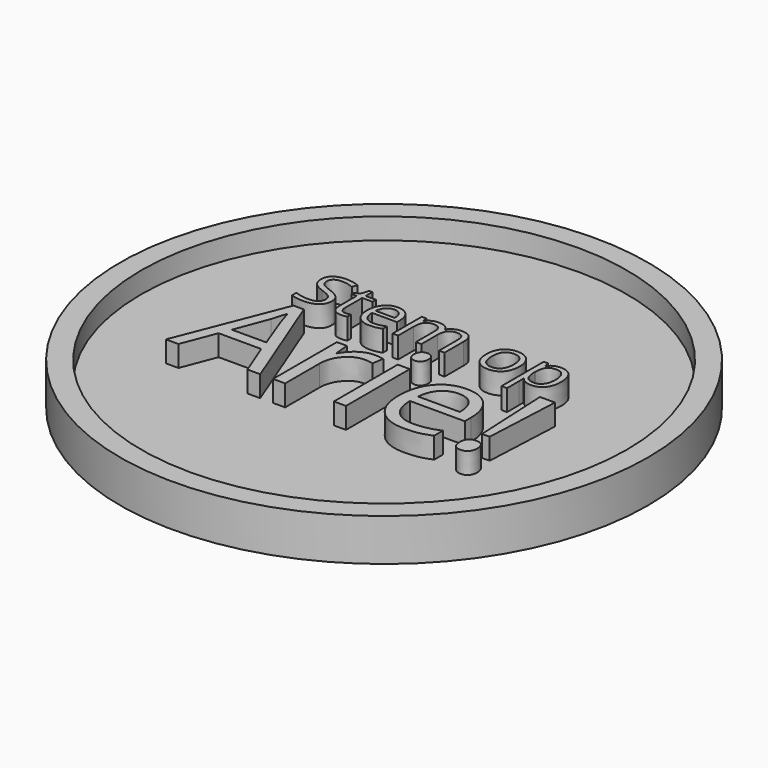
from build123d import *

# Parameters (mm, degrees)
F0_R           = 25
F0_R_2         = 23
F0_TEXT_SIZE   = 6.4365281206
F0_TEXT_SIZE_2 = 14.1188372961
F1_DEPTH       = 4
F0_W           = 1.144949462
F0_H           = 7.5557840218
F2_DEPTH       = 2


# Not quite as in the source:
# - Text() gives the source's letters only with a copy of the font that has no kerning and outlines rounded to 1/6400 em; it was checked with that copy


with BuildPart() as f1:
    # F0 (on Top) → F1 (new body)
    with BuildSketch(Plane.XY):
        with Locations((-25.1149237156, 15.8463213593)):
            Circle(F0_R)
        with Locations((-25.1149237156, 15.8463213593)):
            Circle(F0_R_2, mode=Mode.SUBTRACT)
        with Locations((-37.2358597815, 19.5541195571)):
            Text('Stem op', F0_TEXT_SIZE, font='Open Sans', text_align=(TextAlign.LEFT, TextAlign.BOTTOM))
        with Locations((-39.7772528231, 8.3421012387)):
            Text('Arie!', F0_TEXT_SIZE_2, font='Open Sans', text_align=(TextAlign.LEFT, TextAlign.BOTTOM))
    extrude(amount=F1_DEPTH)

    # F0 (on Top) → F2 (join)
    with BuildSketch(Plane.XY):
        with Locations((-25.1149237156, 15.8463213593)):
            Circle(F0_R_2)
        Polygon((-30.8426760967, 8.3421012387), (-32.0560136768, 8.3421012387), (-33.3112665552, 11.5475185186), (-37.3505776628, 11.5475185186), (-38.5903880629, 8.3421012387), (-39.7772528231, 8.3421012387), (-35.7930934236, 18.4635427253), (-34.8069808812, 18.4635427253), align=None, mode=Mode.SUBTRACT)
        with BuildLine():
            add(Edge.make_bspline(
                [(-27.4850401022, 15.6364661636), (-26.8916077221, 16.0368675651), (-26.1812537206, 16.0368675651)],
                knots=[0, 0, 0, 1, 1, 1], degree=2))
            add(Edge.make_bspline(
                [(-26.1812537206, 16.0368675651), (-25.6782701419, 16.0368675651), (-25.2789717746, 15.9530369686)],
                knots=[0, 0, 0, 1, 1, 1], degree=2))
            Line((-25.2789717746, 15.9530369686), (-25.4378086942, 14.8919181031))
            add(Edge.make_bspline(
                [(-25.4378086942, 14.8919181031), (-25.9054951797, 14.9956033145), (-26.265084317, 14.9956033145)],
                knots=[0, 0, 0, 1, 1, 1], degree=2))
            add(Edge.make_bspline(
                [(-26.265084317, 14.9956033145), (-27.1828087413, 14.9956033145), (-27.8335988979, 14.2510552539)],
                knots=[0, 0, 0, 1, 1, 1], degree=2))
            add(Edge.make_bspline(
                [(-27.8335988979, 14.2510552539), (-28.4843890545, 13.5065071934), (-28.4843890545, 12.3968548247)],
                knots=[0, 0, 0, 1, 1, 1], degree=2))
            Line((-28.4843890545, 12.3968548247), (-28.4843890545, 8.3421012387))
            Line((-28.4843890545, 8.3421012387), (-29.6293385165, 8.3421012387))
            Line((-29.6293385165, 8.3421012387), (-29.6293385165, 15.8978852604))
            Line((-29.6293385165, 15.8978852604), (-28.6851412723, 15.8978852604))
            Line((-28.6851412723, 15.8978852604), (-28.5527771727, 14.4992379408))
            Line((-28.5527771727, 14.4992379408), (-28.4976254645, 14.4992379408))
            add(Edge.make_bspline(
                [(-28.4976254645, 14.4992379408), (-28.0784724823, 15.2360647622), (-27.4850401022, 15.6364661636)],
                knots=[0, 0, 0, 1, 1, 1], degree=2))
        make_face(mode=Mode.SUBTRACT)
        with Locations((-23.2924072457, 12.1199932495)):
            Rectangle(F0_W, F0_H, mode=Mode.SUBTRACT)
        with BuildLine():
            add(Edge.make_bspline(
                [(-15.7950840346, 8.3178344871), (-16.3355707749, 8.203118934), (-17.1010764845, 8.203118934)],
                knots=[0, 0, 0, 1, 1, 1], degree=2))
            add(Edge.make_bspline(
                [(-17.1010764845, 8.203118934), (-18.7754823451, 8.203118934), (-19.7450493751, 9.2245285697)],
                knots=[0, 0, 0, 1, 1, 1], degree=2))
            add(Edge.make_bspline(
                [(-19.7450493751, 9.2245285697), (-20.714616405, 10.2459382053), (-20.714616405, 12.0571203022)],
                knots=[0, 0, 0, 1, 1, 1], degree=2))
            add(Edge.make_bspline(
                [(-20.714616405, 12.0571203022), (-20.714616405, 13.8859509457), (-19.8145405274, 14.9614092554)],
                knots=[0, 0, 0, 1, 1, 1], degree=2))
            add(Edge.make_bspline(
                [(-19.8145405274, 14.9614092554), (-18.9144646497, 16.0368675651), (-17.3966896404, 16.0368675651)],
                knots=[0, 0, 0, 1, 1, 1], degree=2))
            add(Edge.make_bspline(
                [(-17.3966896404, 16.0368675651), (-15.9781877058, 16.0368675651), (-15.150912083, 15.1025976284)],
                knots=[0, 0, 0, 1, 1, 1], degree=2))
            add(Edge.make_bspline(
                [(-15.150912083, 15.1025976284), (-14.3236364602, 14.1683276917), (-14.3236364602, 12.6373162724)],
                knots=[0, 0, 0, 1, 1, 1], degree=2))
            Line((-14.3236364602, 12.6373162724), (-14.3236364602, 11.9137258609))
            Line((-14.3236364602, 11.9137258609), (-19.5277516448, 11.9137258609))
            add(Edge.make_bspline(
                [(-19.5277516448, 11.9137258609), (-19.4924545516, 10.5834666594), (-18.8549008049, 9.8940703071)],
                knots=[0, 0, 0, 1, 1, 1], degree=2))
            add(Edge.make_bspline(
                [(-18.8549008049, 9.8940703071), (-18.2173470583, 9.2046739547), (-17.0591611863, 9.2046739547)],
                knots=[0, 0, 0, 1, 1, 1], degree=2))
            add(Edge.make_bspline(
                [(-17.0591611863, 9.2046739547), (-15.8392054012, 9.2046739547), (-14.6479285043, 9.7142757384)],
                knots=[0, 0, 0, 1, 1, 1], degree=2))
            Line((-14.6479285043, 9.7142757384), (-14.6479285043, 8.6928661027))
            add(Edge.make_bspline(
                [(-14.6479285043, 8.6928661027), (-15.2545972944, 8.4325500401), (-15.7950840346, 8.3178344871)],
                knots=[0, 0, 0, 1, 1, 1], degree=2))
        make_face(mode=Mode.SUBTRACT)
        with BuildLine():
            add(Edge.make_bspline(
                [(-12.301774838, 8.3586467511), (-12.5367211149, 8.5759444814), (-12.5367211149, 9.0723098551)],
                knots=[0, 0, 0, 1, 1, 1], degree=2))
            add(Edge.make_bspline(
                [(-12.5367211149, 9.0723098551), (-12.5367211149, 10.0098888943), (-11.7094454921, 10.0098888943)],
                knots=[0, 0, 0, 1, 1, 1], degree=2))
            add(Edge.make_bspline(
                [(-11.7094454921, 10.0098888943), (-11.3101471248, 10.0098888943), (-11.0928493945, 9.7694274466)],
                knots=[0, 0, 0, 1, 1, 1], degree=2))
            add(Edge.make_bspline(
                [(-11.0928493945, 9.7694274466), (-10.8755516643, 9.5289659989), (-10.8755516643, 9.0723098551)],
                knots=[0, 0, 0, 1, 1, 1], degree=2))
            add(Edge.make_bspline(
                [(-10.8755516643, 9.0723098551), (-10.8755516643, 8.6310961896), (-11.096158497, 8.3862226052)],
                knots=[0, 0, 0, 1, 1, 1], degree=2))
            add(Edge.make_bspline(
                [(-11.096158497, 8.3862226052), (-11.3167653298, 8.1413490209), (-11.7094454921, 8.1413490209)],
                knots=[0, 0, 0, 1, 1, 1], degree=2))
            add(Edge.make_bspline(
                [(-11.7094454921, 8.1413490209), (-12.0668285611, 8.1413490209), (-12.301774838, 8.3586467511)],
                knots=[0, 0, 0, 1, 1, 1], degree=2))
        make_face(mode=Mode.SUBTRACT)
        Polygon((-10.9858550806, 18.4216274271), (-11.3366199447, 11.119541263), (-12.0602103561, 11.119541263), (-12.4131812885, 18.4216274271), align=None, mode=Mode.SUBTRACT)
        with BuildLine():
            add(Edge.make_bspline(
                [(-34.2831025062, 21.5434090294), (-34.0115614761, 21.2477310189), (-34.0115614761, 20.7770599001)],
                knots=[0, 0, 0, 1, 1, 1], degree=2))
            add(Edge.make_bspline(
                [(-34.0115614761, 20.7770599001), (-34.0115614761, 20.1706182662), (-34.4515585156, 19.8306891248)],
                knots=[0, 0, 0, 1, 1, 1], degree=2))
            add(Edge.make_bspline(
                [(-34.4515585156, 19.8306891248), (-34.8915555551, 19.4907599835), (-35.6458361942, 19.4907599835)],
                knots=[0, 0, 0, 1, 1, 1], degree=2))
            add(Edge.make_bspline(
                [(-35.6458361942, 19.4907599835), (-36.4624706995, 19.4907599835), (-36.9029705928, 19.7019585624)],
                knots=[0, 0, 0, 1, 1, 1], degree=2))
            Line((-36.9029705928, 19.7019585624), (-36.9029705928, 20.2168808121))
            add(Edge.make_bspline(
                [(-36.9029705928, 20.2168808121), (-36.6193610725, 20.0982073248), (-36.2864718837, 20.028813506)],
                knots=[0, 0, 0, 1, 1, 1], degree=2))
            add(Edge.make_bspline(
                [(-36.2864718837, 20.028813506), (-35.953582695, 19.9594196872), (-35.6267277514, 19.9594196872)],
                knots=[0, 0, 0, 1, 1, 1], degree=2))
            add(Edge.make_bspline(
                [(-35.6267277514, 19.9594196872), (-35.0926970588, 19.9594196872), (-34.8221617363, 20.1620697523)],
                knots=[0, 0, 0, 1, 1, 1], degree=2))
            add(Edge.make_bspline(
                [(-34.8221617363, 20.1620697523), (-34.5516264137, 20.3647198173), (-34.5516264137, 20.7267745241)],
                knots=[0, 0, 0, 1, 1, 1], degree=2))
            add(Edge.make_bspline(
                [(-34.5516264137, 20.7267745241), (-34.5516264137, 20.9651272061), (-34.6476714818, 21.1174918952)],
                knots=[0, 0, 0, 1, 1, 1], degree=2))
            add(Edge.make_bspline(
                [(-34.6476714818, 21.1174918952), (-34.7437165498, 21.2698565843), (-34.9684921803, 21.3990900005)],
                knots=[0, 0, 0, 1, 1, 1], degree=2))
            add(Edge.make_bspline(
                [(-34.9684921803, 21.3990900005), (-35.1932678107, 21.5283234166), (-35.6518704393, 21.6912480347)],
                knots=[0, 0, 0, 1, 1, 1], degree=2))
            add(Edge.make_bspline(
                [(-35.6518704393, 21.6912480347), (-36.2925061288, 21.920549349), (-36.5675671352, 22.2348329486)],
                knots=[0, 0, 0, 1, 1, 1], degree=2))
            add(Edge.make_bspline(
                [(-36.5675671352, 22.2348329486), (-36.8426281416, 22.5491165483), (-36.8426281416, 23.0549874302)],
                knots=[0, 0, 0, 1, 1, 1], degree=2))
            add(Edge.make_bspline(
                [(-36.8426281416, 23.0549874302), (-36.8426281416, 23.5860010002), (-36.4438651104, 23.9002845998)],
                knots=[0, 0, 0, 1, 1, 1], degree=2))
            add(Edge.make_bspline(
                [(-36.4438651104, 23.9002845998), (-36.0451020792, 24.2145681995), (-35.3873693619, 24.2145681995)],
                knots=[0, 0, 0, 1, 1, 1], degree=2))
            add(Edge.make_bspline(
                [(-35.3873693619, 24.2145681995), (-34.7024825415, 24.2145681995), (-34.1272178408, 23.9631413198)],
                knots=[0, 0, 0, 1, 1, 1], degree=2))
            Line((-34.1272178408, 23.9631413198), (-34.2941652889, 23.498504446))
            add(Edge.make_bspline(
                [(-34.2941652889, 23.498504446), (-34.8633957445, 23.736857128), (-35.4004435596, 23.736857128)],
                knots=[0, 0, 0, 1, 1, 1], degree=2))
            add(Edge.make_bspline(
                [(-35.4004435596, 23.736857128), (-35.8248521326, 23.736857128), (-36.0637076683, 23.5548240671)],
                knots=[0, 0, 0, 1, 1, 1], degree=2))
            add(Edge.make_bspline(
                [(-36.0637076683, 23.5548240671), (-36.302563204, 23.3727910062), (-36.302563204, 23.0489531851)],
                knots=[0, 0, 0, 1, 1, 1], degree=2))
            add(Edge.make_bspline(
                [(-36.302563204, 23.0489531851), (-36.302563204, 22.8106005032), (-36.2145637961, 22.6577329603)],
                knots=[0, 0, 0, 1, 1, 1], degree=2))
            add(Edge.make_bspline(
                [(-36.2145637961, 22.6577329603), (-36.1265643882, 22.5048654174), (-35.9173772243, 22.3776434163)],
                knots=[0, 0, 0, 1, 1, 1], degree=2))
            add(Edge.make_bspline(
                [(-35.9173772243, 22.3776434163), (-35.7081900604, 22.2504214152), (-35.2777472423, 22.0965481648)],
                knots=[0, 0, 0, 1, 1, 1], degree=2))
            add(Edge.make_bspline(
                [(-35.2777472423, 22.0965481648), (-34.5546435363, 21.83908704), (-34.2831025062, 21.5434090294)],
                knots=[0, 0, 0, 1, 1, 1], degree=2))
        make_face(mode=Mode.SUBTRACT)
        with BuildLine():
            add(Edge.make_bspline(
                [(-32.4426577467, 20.0886531034), (-32.2948187414, 19.922208509), (-32.0373576166, 19.922208509)],
                knots=[0, 0, 0, 1, 1, 1], degree=2))
            add(Edge.make_bspline(
                [(-32.0373576166, 19.922208509), (-31.898569979, 19.922208509), (-31.7698394166, 19.9423226594)],
                knots=[0, 0, 0, 1, 1, 1], degree=2))
            add(Edge.make_bspline(
                [(-31.7698394166, 19.9423226594), (-31.6411088542, 19.9624368098), (-31.5656807903, 19.9845623752)],
                knots=[0, 0, 0, 1, 1, 1], degree=2))
            Line((-31.5656807903, 19.9845623752), (-31.5656807903, 19.5852964902))
            add(Edge.make_bspline(
                [(-31.5656807903, 19.5852964902), (-31.6501602218, 19.5450681895), (-31.8150962549, 19.5179140865)],
                knots=[0, 0, 0, 1, 1, 1], degree=2))
            add(Edge.make_bspline(
                [(-31.8150962549, 19.5179140865), (-31.980032288, 19.4907599835), (-32.1127856805, 19.4907599835)],
                knots=[0, 0, 0, 1, 1, 1], degree=2))
            add(Edge.make_bspline(
                [(-32.1127856805, 19.4907599835), (-33.1114532467, 19.4907599835), (-33.1114532467, 20.5437357557)],
                knots=[0, 0, 0, 1, 1, 1], degree=2))
            Line((-33.1114532467, 20.5437357557), (-33.1114532467, 22.5933676791))
            Line((-33.1114532467, 22.5933676791), (-33.6052556385, 22.5933676791))
            Line((-33.6052556385, 22.5933676791), (-33.6052556385, 22.8447945588))
            Line((-33.6052556385, 22.8447945588), (-33.1114532467, 23.0620273829))
            Line((-33.1114532467, 23.0620273829), (-32.8922090076, 23.7971995791))
            Line((-32.8922090076, 23.7971995791), (-32.590496752, 23.7971995791))
            Line((-32.590496752, 23.7971995791), (-32.590496752, 22.9986678092))
            Line((-32.590496752, 22.9986678092), (-31.5908234782, 22.9986678092))
            Line((-31.5908234782, 22.9986678092), (-31.5908234782, 22.5933676791))
            Line((-31.5908234782, 22.5933676791), (-32.590496752, 22.5933676791))
            Line((-32.590496752, 22.5933676791), (-32.590496752, 20.5658613211))
            add(Edge.make_bspline(
                [(-32.590496752, 20.5658613211), (-32.590496752, 20.2550976978), (-32.4426577467, 20.0886531034)],
                knots=[0, 0, 0, 1, 1, 1], degree=2))
        make_face(mode=Mode.SUBTRACT)
        with BuildLine():
            add(Edge.make_bspline(
                [(-28.8271392164, 19.5430567744), (-29.0735375586, 19.4907599835), (-29.4225180676, 19.4907599835)],
                knots=[0, 0, 0, 1, 1, 1], degree=2))
            add(Edge.make_bspline(
                [(-29.4225180676, 19.4907599835), (-30.1858500744, 19.4907599835), (-30.6278585289, 19.9564025647)],
                knots=[0, 0, 0, 1, 1, 1], degree=2))
            add(Edge.make_bspline(
                [(-30.6278585289, 19.9564025647), (-31.0698669835, 20.4220451459), (-31.0698669835, 21.2477310189)],
                knots=[0, 0, 0, 1, 1, 1], degree=2))
            add(Edge.make_bspline(
                [(-31.0698669835, 21.2477310189), (-31.0698669835, 22.081462552), (-30.6595383158, 22.5717449674)],
                knots=[0, 0, 0, 1, 1, 1], degree=2))
            add(Edge.make_bspline(
                [(-30.6595383158, 22.5717449674), (-30.2492096481, 23.0620273829), (-29.5572828751, 23.0620273829)],
                knots=[0, 0, 0, 1, 1, 1], degree=2))
            add(Edge.make_bspline(
                [(-29.5572828751, 23.0620273829), (-28.9106129405, 23.0620273829), (-28.5334726209, 22.6361102486)],
                knots=[0, 0, 0, 1, 1, 1], degree=2))
            add(Edge.make_bspline(
                [(-28.5334726209, 22.6361102486), (-28.1563323014, 22.2101931144), (-28.1563323014, 21.5122320963)],
                knots=[0, 0, 0, 1, 1, 1], degree=2))
            Line((-28.1563323014, 21.5122320963), (-28.1563323014, 21.1823600302))
            Line((-28.1563323014, 21.1823600302), (-30.5287963383, 21.1823600302))
            add(Edge.make_bspline(
                [(-30.5287963383, 21.1823600302), (-30.512705018, 20.5759183963), (-30.2220555451, 20.2616347966)],
                knots=[0, 0, 0, 1, 1, 1], degree=2))
            add(Edge.make_bspline(
                [(-30.2220555451, 20.2616347966), (-29.9314060721, 19.947351197), (-29.4034096247, 19.947351197)],
                knots=[0, 0, 0, 1, 1, 1], degree=2))
            add(Edge.make_bspline(
                [(-29.4034096247, 19.947351197), (-28.8472533668, 19.947351197), (-28.3041713066, 20.1796696339)],
                knots=[0, 0, 0, 1, 1, 1], degree=2))
            Line((-28.3041713066, 20.1796696339), (-28.3041713066, 19.7140270526))
            add(Edge.make_bspline(
                [(-28.3041713066, 19.7140270526), (-28.5807408743, 19.5953535654), (-28.8271392164, 19.5430567744)],
                knots=[0, 0, 0, 1, 1, 1], degree=2))
        make_face(mode=Mode.SUBTRACT)
        with BuildLine():
            add(Edge.make_bspline(
                [(-23.7689180045, 17.3693328349), (-23.9619489831, 17.5590547111), (-23.9619489831, 17.9451166684)],
                knots=[0, 0, 0, 1, 1, 1], degree=2))
            add(Edge.make_bspline(
                [(-23.9619489831, 17.9451166684), (-23.9619489831, 18.3377968307), (-23.7689180045, 18.5209005019)],
                knots=[0, 0, 0, 1, 1, 1], degree=2))
            add(Edge.make_bspline(
                [(-23.7689180045, 18.5209005019), (-23.5758870258, 18.704004173), (-23.2846860066, 18.704004173)],
                knots=[0, 0, 0, 1, 1, 1], degree=2))
            add(Edge.make_bspline(
                [(-23.2846860066, 18.704004173), (-23.0089274656, 18.704004173), (-22.809278282, 18.5175913994)],
                knots=[0, 0, 0, 1, 1, 1], degree=2))
            add(Edge.make_bspline(
                [(-22.809278282, 18.5175913994), (-22.6096290983, 18.3311786257), (-22.6096290983, 17.9451166684)],
                knots=[0, 0, 0, 1, 1, 1], degree=2))
            add(Edge.make_bspline(
                [(-22.6096290983, 17.9451166684), (-22.6096290983, 17.5590547111), (-22.809278282, 17.3693328349)],
                knots=[0, 0, 0, 1, 1, 1], degree=2))
            add(Edge.make_bspline(
                [(-22.809278282, 17.3693328349), (-23.0089274656, 17.1796109587), (-23.2846860066, 17.1796109587)],
                knots=[0, 0, 0, 1, 1, 1], degree=2))
            add(Edge.make_bspline(
                [(-23.2846860066, 17.1796109587), (-23.5758870258, 17.1796109587), (-23.7689180045, 17.3693328349)],
                knots=[0, 0, 0, 1, 1, 1], degree=2))
        make_face(mode=Mode.SUBTRACT)
        with BuildLine():
            Line((-22.3544056252, 19.5541195571), (-22.8753621199, 19.5541195571))
            Line((-22.8753621199, 19.5541195571), (-22.8753621199, 21.7948359091))
            add(Edge.make_bspline(
                [(-22.8753621199, 21.7948359091), (-22.8753621199, 22.2071759919), (-23.0513609357, 22.4128431795)],
                knots=[0, 0, 0, 1, 1, 1], degree=2))
            add(Edge.make_bspline(
                [(-23.0513609357, 22.4128431795), (-23.2273597515, 22.6185103671), (-23.598465826, 22.6185103671)],
                knots=[0, 0, 0, 1, 1, 1], degree=2))
            add(Edge.make_bspline(
                [(-23.598465826, 22.6185103671), (-24.0852282651, 22.6185103671), (-24.3180495557, 22.3389236768)],
                knots=[0, 0, 0, 1, 1, 1], degree=2))
            add(Edge.make_bspline(
                [(-24.3180495557, 22.3389236768), (-24.5508708463, 22.0593369866), (-24.5508708463, 21.4780380407)],
                knots=[0, 0, 0, 1, 1, 1], degree=2))
            Line((-24.5508708463, 21.4780380407), (-24.5508708463, 19.5541195571))
            Line((-24.5508708463, 19.5541195571), (-25.0728330486, 19.5541195571))
            Line((-25.0728330486, 19.5541195571), (-25.0728330486, 21.7948359091))
            add(Edge.make_bspline(
                [(-25.0728330486, 21.7948359091), (-25.0728330486, 22.2071759919), (-25.2488318644, 22.4128431795)],
                knots=[0, 0, 0, 1, 1, 1], degree=2))
            add(Edge.make_bspline(
                [(-25.2488318644, 22.4128431795), (-25.4248306802, 22.6185103671), (-25.7989538772, 22.6185103671)],
                knots=[0, 0, 0, 1, 1, 1], degree=2))
            add(Edge.make_bspline(
                [(-25.7989538772, 22.6185103671), (-26.2887334389, 22.6185103671), (-26.5165261919, 22.3248437716)],
                knots=[0, 0, 0, 1, 1, 1], degree=2))
            add(Edge.make_bspline(
                [(-26.5165261919, 22.3248437716), (-26.7443189449, 22.0311771761), (-26.7443189449, 21.3613759685)],
                knots=[0, 0, 0, 1, 1, 1], degree=2))
            Line((-26.7443189449, 21.3613759685), (-26.7443189449, 19.5541195571))
            Line((-26.7443189449, 19.5541195571), (-27.2662811472, 19.5541195571))
            Line((-27.2662811472, 19.5541195571), (-27.2662811472, 22.9986678092))
            Line((-27.2662811472, 22.9986678092), (-26.8418725742, 22.9986678092))
            Line((-26.8418725742, 22.9986678092), (-26.7573931427, 22.5269909828))
            Line((-26.7573931427, 22.5269909828), (-26.7322504547, 22.5269909828))
            add(Edge.make_bspline(
                [(-26.7322504547, 22.5269909828), (-26.5844114494, 22.7784178626), (-26.3153846881, 22.9202226227)],
                knots=[0, 0, 0, 1, 1, 1], degree=2))
            add(Edge.make_bspline(
                [(-26.3153846881, 22.9202226227), (-26.0463579268, 23.0620273829), (-25.7134687381, 23.0620273829)],
                knots=[0, 0, 0, 1, 1, 1], degree=2))
            add(Edge.make_bspline(
                [(-25.7134687381, 23.0620273829), (-24.9058856005, 23.0620273829), (-24.6574758433, 22.4767056069)],
                knots=[0, 0, 0, 1, 1, 1], degree=2))
            Line((-24.6574758433, 22.4767056069), (-24.6323331553, 22.4767056069))
            add(Edge.make_bspline(
                [(-24.6323331553, 22.4767056069), (-24.478459905, 22.7472409295), (-24.1863018707, 22.9046341562)],
                knots=[0, 0, 0, 1, 1, 1], degree=2))
            add(Edge.make_bspline(
                [(-24.1863018707, 22.9046341562), (-23.8941438365, 23.0620273829), (-23.5200206395, 23.0620273829)],
                knots=[0, 0, 0, 1, 1, 1], degree=2))
            add(Edge.make_bspline(
                [(-23.5200206395, 23.0620273829), (-22.9357045711, 23.0620273829), (-22.6450550981, 22.7618236885)],
                knots=[0, 0, 0, 1, 1, 1], degree=2))
            add(Edge.make_bspline(
                [(-22.6450550981, 22.7618236885), (-22.3544056252, 22.4616199941), (-22.3544056252, 21.8008701542)],
                knots=[0, 0, 0, 1, 1, 1], degree=2))
            Line((-22.3544056252, 21.8008701542), (-22.3544056252, 19.5541195571))
        make_face(mode=Mode.SUBTRACT)
        with BuildLine():
            add(Edge.make_bspline(
                [(-17.0598583922, 22.5807963351), (-16.633941258, 22.0995652873), (-16.633941258, 21.2799136595)],
                knots=[0, 0, 0, 1, 1, 1], degree=2))
            add(Edge.make_bspline(
                [(-16.633941258, 21.2799136595), (-16.633941258, 20.4371307587), (-17.0578469772, 19.9639453711)],
                knots=[0, 0, 0, 1, 1, 1], degree=2))
            add(Edge.make_bspline(
                [(-17.0578469772, 19.9639453711), (-17.4817526964, 19.4907599835), (-18.2299990904, 19.4907599835)],
                knots=[0, 0, 0, 1, 1, 1], degree=2))
            add(Edge.make_bspline(
                [(-18.2299990904, 19.4907599835), (-18.6926245491, 19.4907599835), (-19.0506564258, 19.7079928075)],
                knots=[0, 0, 0, 1, 1, 1], degree=2))
            add(Edge.make_bspline(
                [(-19.0506564258, 19.7079928075), (-19.4086883025, 19.9252256316), (-19.6037955611, 20.3305257617)],
                knots=[0, 0, 0, 1, 1, 1], degree=2))
            add(Edge.make_bspline(
                [(-19.6037955611, 20.3305257617), (-19.7989028198, 20.7358258918), (-19.7989028198, 21.2799136595)],
                knots=[0, 0, 0, 1, 1, 1], degree=2))
            add(Edge.make_bspline(
                [(-19.7989028198, 21.2799136595), (-19.7989028198, 22.1216908528), (-19.3775113694, 22.5918591178)],
                knots=[0, 0, 0, 1, 1, 1], degree=2))
            add(Edge.make_bspline(
                [(-19.3775113694, 22.5918591178), (-18.956119919, 23.0620273829), (-18.207873525, 23.0620273829)],
                knots=[0, 0, 0, 1, 1, 1], degree=2))
            add(Edge.make_bspline(
                [(-18.207873525, 23.0620273829), (-17.4857755264, 23.0620273829), (-17.0598583922, 22.5807963351)],
                knots=[0, 0, 0, 1, 1, 1], degree=2))
        make_face(mode=Mode.SUBTRACT)
        with BuildLine():
            add(Edge.make_bspline(
                [(-13.0641824198, 19.9609282485), (-13.4428313007, 19.4907599835), (-14.1156496308, 19.4907599835)],
                knots=[0, 0, 0, 1, 1, 1], degree=2))
            add(Edge.make_bspline(
                [(-14.1156496308, 19.4907599835), (-14.4525616496, 19.4907599835), (-14.7306397786, 19.614964862)],
                knots=[0, 0, 0, 1, 1, 1], degree=2))
            add(Edge.make_bspline(
                [(-14.7306397786, 19.614964862), (-15.0087179075, 19.7391697406), (-15.1967852135, 19.997636573)],
                knots=[0, 0, 0, 1, 1, 1], degree=2))
            Line((-15.1967852135, 19.997636573), (-15.2350020993, 19.997636573))
            add(Edge.make_bspline(
                [(-15.2350020993, 19.997636573), (-15.1967852135, 19.6959243173), (-15.1967852135, 19.4253889947)],
                knots=[0, 0, 0, 1, 1, 1], degree=2))
            Line((-15.1967852135, 19.4253889947), (-15.1967852135, 18.0073413932))
            Line((-15.1967852135, 18.0073413932), (-15.7187474158, 18.0073413932))
            Line((-15.7187474158, 18.0073413932), (-15.7187474158, 22.9986678092))
            Line((-15.7187474158, 22.9986678092), (-15.2943388429, 22.9986678092))
            Line((-15.2943388429, 22.9986678092), (-15.2219279015, 22.5269909828))
            Line((-15.2219279015, 22.5269909828), (-15.1967852135, 22.5269909828))
            add(Edge.make_bspline(
                [(-15.1967852135, 22.5269909828), (-14.9956437098, 22.8106005032), (-14.7286283635, 22.936313943)],
                knots=[0, 0, 0, 1, 1, 1], degree=2))
            add(Edge.make_bspline(
                [(-14.7286283635, 22.936313943), (-14.4616130173, 23.0620273829), (-14.1156496308, 23.0620273829)],
                knots=[0, 0, 0, 1, 1, 1], degree=2))
            add(Edge.make_bspline(
                [(-14.1156496308, 23.0620273829), (-13.4307628105, 23.0620273829), (-13.0581481747, 22.5933676791)],
                knots=[0, 0, 0, 1, 1, 1], degree=2))
            add(Edge.make_bspline(
                [(-13.0581481747, 22.5933676791), (-12.685533539, 22.1247079753), (-12.685533539, 21.2799136595)],
                knots=[0, 0, 0, 1, 1, 1], degree=2))
            add(Edge.make_bspline(
                [(-12.685533539, 21.2799136595), (-12.685533539, 20.4310965136), (-13.0641824198, 19.9609282485)],
                knots=[0, 0, 0, 1, 1, 1], degree=2))
        make_face(mode=Mode.SUBTRACT)
        with BuildLine():
            Line((-36.9358368173, 12.6020191791), (-33.6752678292, 12.6020191791))
            Line((-33.6752678292, 12.6020191791), (-34.8488961794, 15.7258119309))
            add(Edge.make_bspline(
                [(-34.8488961794, 15.7258119309), (-35.0761212172, 16.319244311), (-35.3165826649, 17.1796109587)],
                knots=[0, 0, 0, 1, 1, 1], degree=2))
            add(Edge.make_bspline(
                [(-35.3165826649, 17.1796109587), (-35.4688013795, 16.5177904605), (-35.7511781254, 15.7258119309)],
                knots=[0, 0, 0, 1, 1, 1], degree=2))
            Line((-35.7511781254, 15.7258119309), (-36.9358368173, 12.6020191791))
        make_face()
        with BuildLine():
            add(Edge.make_bspline(
                [(-16.0322363798, 14.5014440091), (-16.5142623094, 15.0772278426), (-17.4121321187, 15.0772278426)],
                knots=[0, 0, 0, 1, 1, 1], degree=2))
            add(Edge.make_bspline(
                [(-17.4121321187, 15.0772278426), (-18.3210322696, 15.0772278426), (-18.8626220441, 14.4848984967)],
                knots=[0, 0, 0, 1, 1, 1], degree=2))
            add(Edge.make_bspline(
                [(-18.8626220441, 14.4848984967), (-19.4042118185, 13.8925691507), (-19.5012788249, 12.8446866951)],
                knots=[0, 0, 0, 1, 1, 1], degree=2))
            Line((-19.5012788249, 12.8446866951), (-15.5502104503, 12.8446866951))
            add(Edge.make_bspline(
                [(-15.5502104503, 12.8446866951), (-15.5502104503, 13.9256601756), (-16.0322363798, 14.5014440091)],
                knots=[0, 0, 0, 1, 1, 1], degree=2))
        make_face()
        with BuildLine():
            add(Edge.make_bspline(
                [(-18.9968510735, 22.282101202), (-19.2578321746, 21.945692037), (-19.2578321746, 21.2799136595)],
                knots=[0, 0, 0, 1, 1, 1], degree=2))
            add(Edge.make_bspline(
                [(-19.2578321746, 21.2799136595), (-19.2578321746, 20.6191638196), (-18.9938339509, 20.2737032869)],
                knots=[0, 0, 0, 1, 1, 1], degree=2))
            add(Edge.make_bspline(
                [(-18.9938339509, 20.2737032869), (-18.7298357272, 19.9282427542), (-18.2179306002, 19.9282427542)],
                knots=[0, 0, 0, 1, 1, 1], degree=2))
            add(Edge.make_bspline(
                [(-18.2179306002, 19.9282427542), (-17.7050197655, 19.9282427542), (-17.4395129806, 20.2721947256)],
                knots=[0, 0, 0, 1, 1, 1], degree=2))
            add(Edge.make_bspline(
                [(-17.4395129806, 20.2721947256), (-17.1740061956, 20.616146697), (-17.1740061956, 21.2799136595)],
                knots=[0, 0, 0, 1, 1, 1], degree=2))
            add(Edge.make_bspline(
                [(-17.1740061956, 21.2799136595), (-17.1740061956, 21.9366406693), (-17.4395129806, 22.2775755182)],
                knots=[0, 0, 0, 1, 1, 1], degree=2))
            add(Edge.make_bspline(
                [(-17.4395129806, 22.2775755182), (-17.7050197655, 22.6185103671), (-18.2239648453, 22.6185103671)],
                knots=[0, 0, 0, 1, 1, 1], degree=2))
            add(Edge.make_bspline(
                [(-18.2239648453, 22.6185103671), (-18.7358699724, 22.6185103671), (-18.9968510735, 22.282101202)],
                knots=[0, 0, 0, 1, 1, 1], degree=2))
        make_face()
        with BuildLine():
            add(Edge.make_bspline(
                [(-13.4795396251, 22.2745583956), (-13.7324750661, 22.6185103671), (-14.1910776947, 22.6185103671)],
                knots=[0, 0, 0, 1, 1, 1], degree=2))
            add(Edge.make_bspline(
                [(-14.1910776947, 22.6185103671), (-14.7190741421, 22.6185103671), (-14.9549125553, 22.3263523328)],
                knots=[0, 0, 0, 1, 1, 1], degree=2))
            add(Edge.make_bspline(
                [(-14.9549125553, 22.3263523328), (-15.1907509684, 22.0341942986), (-15.1967852135, 21.3955700241)],
                knots=[0, 0, 0, 1, 1, 1], degree=2))
            Line((-15.1967852135, 21.3955700241), (-15.1967852135, 21.2799136595))
            add(Edge.make_bspline(
                [(-15.1967852135, 21.2799136595), (-15.1967852135, 20.5537928309), (-14.9549125553, 20.2410177925)],
                knots=[0, 0, 0, 1, 1, 1], degree=2))
            add(Edge.make_bspline(
                [(-14.9549125553, 20.2410177925), (-14.713039897, 19.9282427542), (-14.1790092045, 19.9282427542)],
                knots=[0, 0, 0, 1, 1, 1], degree=2))
            add(Edge.make_bspline(
                [(-14.1790092045, 19.9282427542), (-13.7324750661, 19.9282427542), (-13.4795396251, 20.2897946072)],
                knots=[0, 0, 0, 1, 1, 1], degree=2))
            add(Edge.make_bspline(
                [(-13.4795396251, 20.2897946072), (-13.2266041841, 20.6513464602), (-13.2266041841, 21.2859479046)],
                knots=[0, 0, 0, 1, 1, 1], degree=2))
            add(Edge.make_bspline(
                [(-13.2266041841, 21.2859479046), (-13.2266041841, 21.9306064242), (-13.4795396251, 22.2745583956)],
                knots=[0, 0, 0, 1, 1, 1], degree=2))
        make_face()
        with BuildLine():
            add(Edge.make_bspline(
                [(-28.9352527747, 22.3620549498), (-29.1549998676, 22.6245446122), (-29.5643228278, 22.6245446122)],
                knots=[0, 0, 0, 1, 1, 1], degree=2))
            add(Edge.make_bspline(
                [(-29.5643228278, 22.6245446122), (-29.9786743255, 22.6245446122), (-30.2255755214, 22.3545121434)],
                knots=[0, 0, 0, 1, 1, 1], degree=2))
            add(Edge.make_bspline(
                [(-30.2255755214, 22.3545121434), (-30.4724767173, 22.0844796746), (-30.5167278481, 21.6067686031)],
                knots=[0, 0, 0, 1, 1, 1], degree=2))
            Line((-30.5167278481, 21.6067686031), (-28.7155056819, 21.6067686031))
            add(Edge.make_bspline(
                [(-28.7155056819, 21.6067686031), (-28.7155056819, 22.0995652873), (-28.9352527747, 22.3620549498)],
                knots=[0, 0, 0, 1, 1, 1], degree=2))
        make_face()
    extrude(amount=F2_DEPTH)


solid = f1.part
